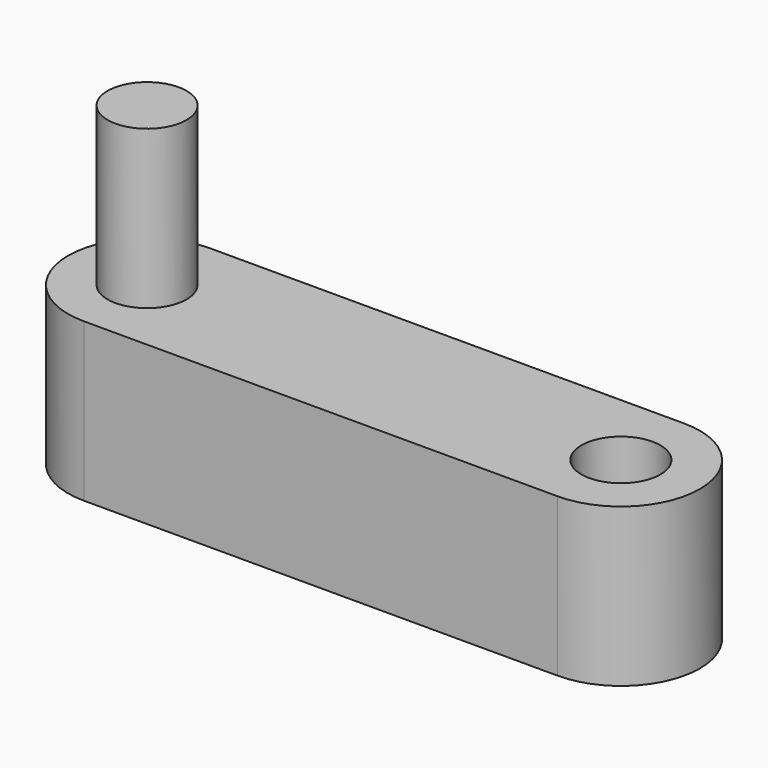
from build123d import *

# Parameters (mm, degrees)
F2_DEPTH = 25.4
F3_R     = 6.35
F4_DEPTH = 25.4
F5_DEPTH = 25.4


# Not quite as in the source:
# - a variable given as a bare number and used for a length is read in inches; the dataset says mm whatever the document's units were


with BuildPart() as f2:
    # F1 (on Top) → F2 (new body)
    with BuildSketch(Plane.XY):
        with BuildLine():
            ThreePointArc((-23.1655191958, -10.2824198201), (-10.4655191958, 2.4175801799), (-23.1655191958, 15.1175801799))
            Line((-23.1655191958, 15.1175801799), (-99.3655191958, 15.1175801799))
            ThreePointArc((-99.3655191958, 15.1175801799), (-112.0655191958, 2.4175801799), (-99.3655191958, -10.2824198201))
            Line((-99.3655191958, -10.2824198201), (-23.1655191958, -10.2824198201))
        make_face()
    extrude(amount=F2_DEPTH)

    # F3 (on face) → F4 (join)
    with BuildSketch(Plane.XY.offset(25.4)):
        with Locations((-99.3655191958, 2.4175801799)):
            Circle(F3_R)
    extrude(amount=F4_DEPTH)

    # F3 (on face) → F5 (cut)
    with BuildSketch(Plane.XY.offset(25.4)):
        with Locations((-23.1655191958, 2.4175801799)):
            Circle(F3_R)
    extrude(amount=-F5_DEPTH, mode=Mode.SUBTRACT)


solid = f2.part
